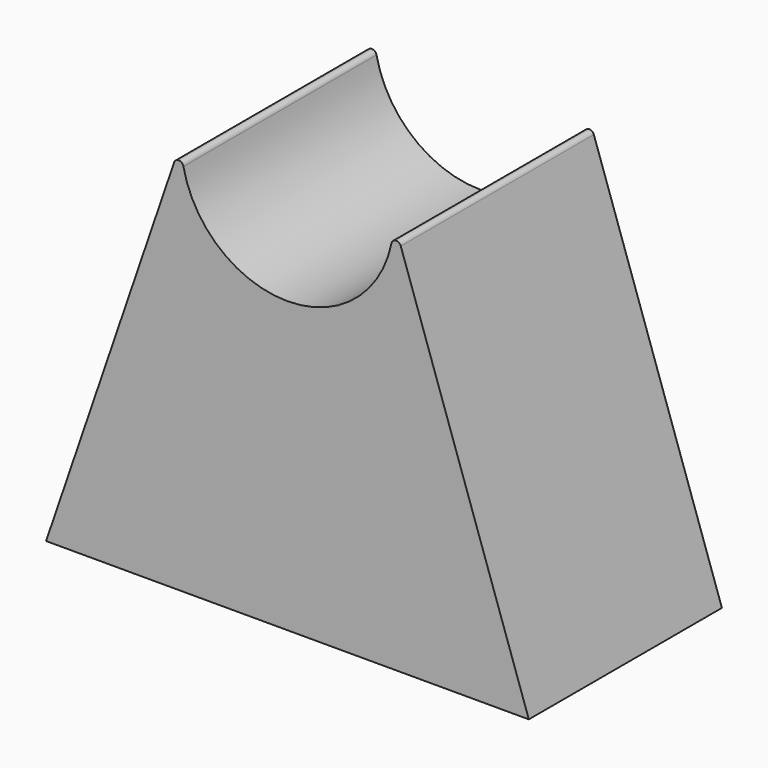
from build123d import *

# Parameters (mm, degrees)
F1_DEPTH = 25
F2_R     = 0.5


with BuildPart() as f1:
    # F0 (on Front) → F1 (new body)
    with BuildSketch(Plane.XZ):
        with BuildLine():
            Line((25, 0), (11, 41))
            ThreePointArc((11, 41), (0, 30), (-11, 41))
            Line((-11, 41), (-25, 0))
            Line((-25, 0), (25, 0))
        make_face()
    extrude(amount=F1_DEPTH)

    # F2
    f2_edges = [f1.edges().sort_by_distance(p)[0] for p in [
        (-11, -12.5, 41),
        (11, -12.5, 41),
    ]]
    fillet(f2_edges, radius=F2_R)


solid = f1.part
